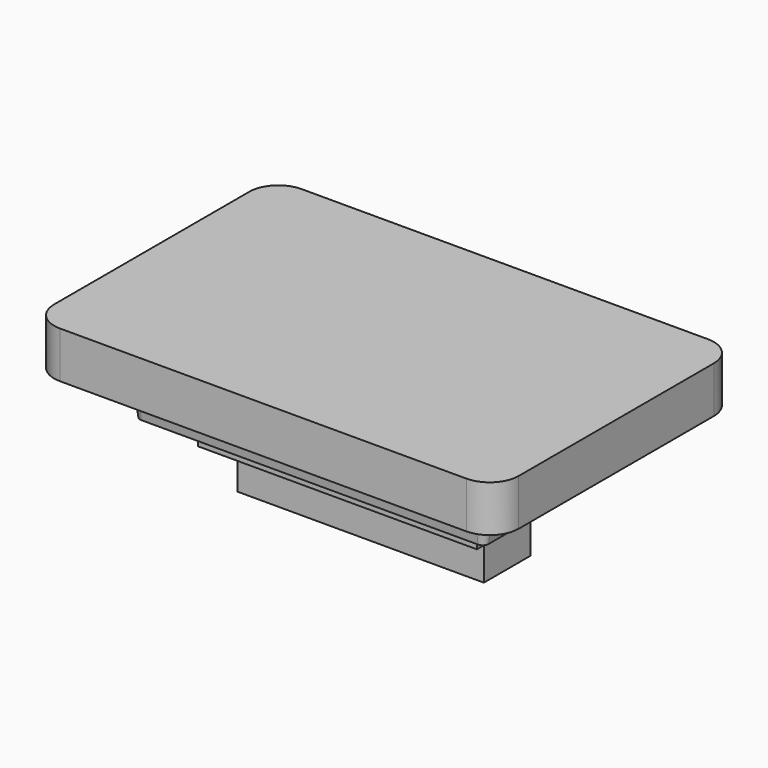
from build123d import *

# Parameters (mm, degrees)
F1_DEPTH = 2.6
F2_W     = 10.6
F2_H     = 2.5
F3_DEPTH = 2
F5_DEPTH = 0.6
F7_DEPTH = 2
F9_DEPTH = 2
F9_TAPER = 7


# Not quite as in the source:
# - a feature names something its author has since deleted; it is built from what else it names


with BuildPart() as f1:
    # F0 (on Top) → F1 (new body)
    with BuildSketch(Plane.XY):
        Polygon((6, 2.5), (-6, 2.5), (-6, 1.25), (-5.3, 1.25), (-5.3, -1.25), (-6, -1.25), (-6, -2.5), (6, -2.5), (6, -1.25), (5.3, -1.25), (5.3, 1.25), (6, 1.25), align=None)
    extrude(amount=F1_DEPTH)

    # F2 (on face) → F3 (join)
    with BuildSketch(Plane(origin=(0, 0, 0), x_dir=(1, 0, 0), z_dir=(0, 0, -1))):
        Rectangle(F2_W, F2_H)
    extrude(amount=F3_DEPTH)

    # F4 (on face) → F5 (join)
    with BuildSketch(Plane.XY.offset(2.6)):
        Polygon((5.375, 1.875), (-5.375, 1.875), (-5.375, 1.25), (-5.3, 1.25), (-5.3, -1.25), (-5.375, -1.25), (-5.375, -1.875), (5.375, -1.875), (5.375, -1.25), (5.3, -1.25), (5.3, 1.25), (5.375, 1.25), align=None)
    extrude(amount=F5_DEPTH)

    # F6 (on face) → F7 (join)
    with BuildSketch(Plane.XY.offset(3.2)):
        with BuildLine():
            Line((8.75, 6.5), (-8.75, 6.5))
            ThreePointArc((-8.75, 6.5), (-9.6338834765, 6.1338834765), (-10, 5.25))
            Line((-10, 5.25), (-10, -5.25))
            ThreePointArc((-10, -5.25), (-9.6338834765, -6.1338834765), (-8.75, -6.5))
            Line((-8.75, -6.5), (8.75, -6.5))
            ThreePointArc((8.75, -6.5), (9.6338834765, -6.1338834765), (10, -5.25))
            Line((10, -5.25), (10, 5.25))
            ThreePointArc((10, 5.25), (9.6338834765, 6.1338834765), (8.75, 6.5))
        make_face()
    extrude(amount=F7_DEPTH)

    # F8 (on face) → F9 (join)
    with BuildSketch(Plane(origin=(0, 0, 3.2), x_dir=(1, 0, 0), z_dir=(0, 0, -1))):
        with BuildLine():
            Line((7.25, 4.25), (-7.25, 4.25))
            ThreePointArc((-7.25, 4.25), (-7.6035533906, 4.1035533906), (-7.75, 3.75))
            Line((-7.75, 3.75), (-7.75, -3.75))
            ThreePointArc((-7.75, -3.75), (-7.6035533906, -4.1035533906), (-7.25, -4.25))
            Line((-7.25, -4.25), (7.25, -4.25))
            ThreePointArc((7.25, -4.25), (7.6035533906, -4.1035533906), (7.75, -3.75))
            Line((7.75, -3.75), (7.75, 3.75))
            ThreePointArc((7.75, 3.75), (7.6035533906, 4.1035533906), (7.25, 4.25))
        make_face()
        with BuildLine():
            ThreePointArc((-6.75, 3), (-6.6035533906, 3.3535533906), (-6.25, 3.5))
            Line((-6.25, 3.5), (6.25, 3.5))
            ThreePointArc((6.25, 3.5), (6.6035533906, 3.3535533906), (6.75, 3))
            Line((6.75, 3), (6.75, -3))
            ThreePointArc((6.75, -3), (6.6035533906, -3.3535533906), (6.25, -3.5))
            Line((6.25, -3.5), (-6.25, -3.5))
            ThreePointArc((-6.25, -3.5), (-6.6035533906, -3.3535533906), (-6.75, -3))
            Line((-6.75, -3), (-6.75, 3))
        make_face(mode=Mode.SUBTRACT)
    extrude(amount=F9_DEPTH, taper=F9_TAPER)


solid = f1.part
